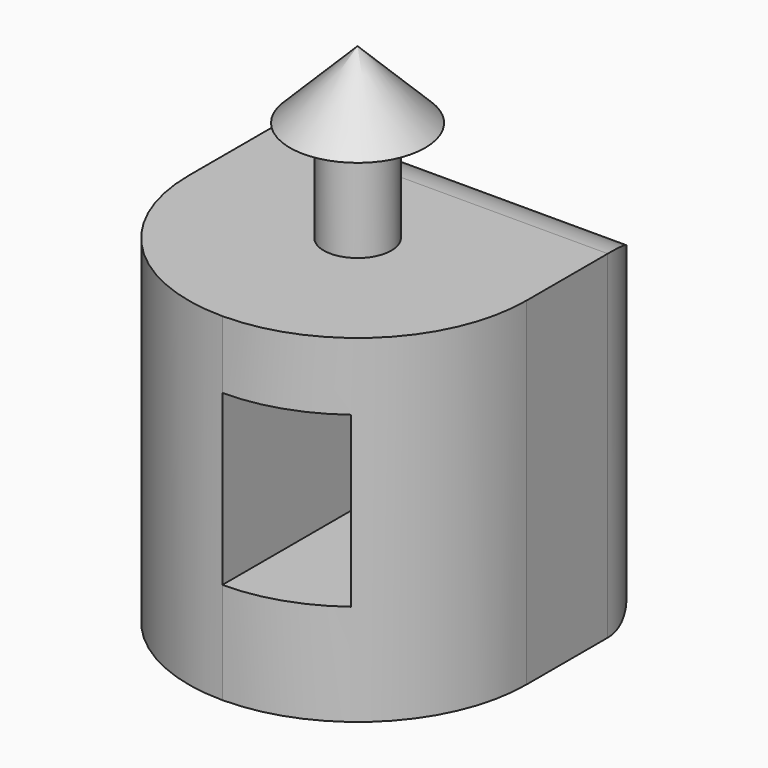
from build123d import *

# Parameters (mm, degrees)
F0_W          = 25.4
F0_H          = 25.4
F1_DEPTH      = 25.4
F2_T1_DEPTH   = 88.9
F3_R          = 2.54
F4_DEPTH      = 7.62
F5_R          = 5.08
F6_DEPTH      = 5.08
F7_SIZE       = 5.07999
F8_W          = 7.62
F8_H          = 12.7
F9_DEPTH      = 25.4
F10_T1_DEPTH  = 50.8
F10_T3_DEPTH  = 50.8
F10_T5_DEPTH  = 7.62
F10_T7_DEPTH  = 12.7
F10_T13_DEPTH = 20.32
F10_T18_DEPTH = 25.4
F10_T26_DEPTH = 20.32
F10_T30_DEPTH = 25.4
F10_T38_DEPTH = 25.4
F10_T43_DEPTH = 20.32
F10_T51_DEPTH = 20.32
F10_T55_DEPTH = 25.4


# Not quite as in the source:
# - a fillet or chamfer that OpenCascade refuses, or shapes differently, is made with other operations: its cross-section is extruded or revolved along the edge and cut away or added
# - a fillet or chamfer is up to 0.001 mm smaller than in the source, because OpenCascade refuses the exact size


with BuildPart() as f1:
    # F0 (on Top) → F1 (new body)
    with BuildSketch(Plane.XY):
        with Locations((12.7, 12.7)):
            Rectangle(F0_W, F0_H)
    extrude(amount=F1_DEPTH)

    # F2: fillet of radius 12.7 on 2 edges, made by hand

    # F2_s2 → F2_t1 (cut)
    with BuildSketch(Plane.XY.offset(-31.75)):
        with BuildLine():
            ThreePointArc((0, 12.7), (3.7197438789, 3.7197438789), (12.7, 0))
            Line((12.7, 0), (0, 0))
            Line((0, 0), (0, 12.7))
        make_face()
        with BuildLine():
            ThreePointArc((12.7, 0), (21.6802561211, 3.7197438789), (25.4, 12.7))
            Line((25.4, 12.7), (25.4, 0))
            Line((25.4, 0), (12.7, 0))
        make_face()
    extrude(amount=F2_T1_DEPTH, mode=Mode.SUBTRACT)

    # F3 (on face) → F4 (join)
    with BuildSketch(Plane.XY.offset(25.4)):
        with Locations((12.7, 12.7)):
            Circle(F3_R)
    extrude(amount=F4_DEPTH)

    # F5 (on face) → F6 (join)
    with BuildSketch(Plane.XY.offset(33.02)):
        with Locations((12.7, 12.7)):
            Circle(F5_R)
    extrude(amount=F6_DEPTH)

    # F7 (size 5.08 in the source; OpenCascade refuses exactly that, so slightly less here)
    f7_edges = [f1.edges().sort_by_distance(p)[0] for p in [
        (7.62, 12.7, 38.1),
    ]]
    chamfer(f7_edges, length=F7_SIZE)

    # F8 (on face) → F9 (cut)
    with BuildSketch(Plane(origin=(0, 25.4, 0), x_dir=(-1, 0, 0), z_dir=(0, 1, 0))):
        with Locations((-16.51, 13.97)):
            Rectangle(F8_W, F8_H)
    extrude(amount=-F9_DEPTH, mode=Mode.SUBTRACT)

    # F10: fillet of radius 5.08 on 8 edges, made by hand

    # F10_s2 → F10_t1 (cut)
    with BuildSketch(Plane.XY.offset(-12.7)):
        with BuildLine():
            ThreePointArc((20.32, 25.4), (23.9121024484, 23.9121024484), (25.4, 20.32))
            Line((25.4, 20.32), (25.4, 25.4))
            Line((25.4, 25.4), (20.32, 25.4))
        make_face()
        with BuildLine():
            ThreePointArc((5.08, 25.4), (1.4878975516, 23.9121024484), (0, 20.32))
            Line((0, 20.32), (0, 25.4))
            Line((0, 25.4), (5.08, 25.4))
        make_face()
    extrude(amount=F10_T1_DEPTH, mode=Mode.SUBTRACT)

    # F10_s4 → F10_t3 (cut)
    with BuildSketch(Plane.YZ.offset(-12.7)):
        with BuildLine():
            ThreePointArc((25.4, 5.08), (23.9121024484, 1.4878975516), (20.32, 0))
            Line((20.32, 0), (25.4, 0))
            Line((25.4, 0), (25.4, 5.08))
        make_face()
        with BuildLine():
            ThreePointArc((20.32, 25.4), (23.9121024484, 23.9121024484), (25.4, 20.32))
            Line((25.4, 20.32), (25.4, 25.4))
            Line((25.4, 25.4), (20.32, 25.4))
        make_face()
    extrude(amount=F10_T3_DEPTH, mode=Mode.SUBTRACT)

    # F10_s6 → F10_t5 (cut)
    with BuildSketch(Plane.YZ.offset(12.7)):
        with BuildLine():
            ThreePointArc((25.4, 2.54), (23.9121024484, 6.1321024484), (20.32, 7.62))
            Line((20.32, 7.62), (25.4, 7.62))
            Line((25.4, 7.62), (25.4, 2.54))
        make_face()
        with BuildLine():
            ThreePointArc((25.4, 25.4), (23.9121024484, 21.8078975516), (20.32, 20.32))
            Line((20.32, 20.32), (25.4, 20.32))
            Line((25.4, 20.32), (25.4, 25.4))
        make_face()
    extrude(amount=F10_T5_DEPTH, mode=Mode.SUBTRACT)

    # F10_s8 → F10_t7 (cut)
    with BuildSketch(Plane.XY.offset(7.62)):
        with BuildLine():
            ThreePointArc((25.4, 25.4), (21.8078975516, 23.9121024484), (20.32, 20.32))
            Line((20.32, 20.32), (20.32, 25.4))
            Line((20.32, 25.4), (25.4, 25.4))
        make_face()
        with BuildLine():
            ThreePointArc((7.62, 25.4), (11.2121024484, 23.9121024484), (12.7, 20.32))
            Line((12.7, 20.32), (12.7, 25.4))
            Line((12.7, 25.4), (7.62, 25.4))
        make_face()
    extrude(amount=F10_T7_DEPTH, mode=Mode.SUBTRACT)


with BuildPart() as f10_tool11:
    # F10_s12 → F10_t13 (new body)
    with BuildSketch(Plane.YZ.offset(33.02)):
        with BuildLine():
            ThreePointArc((25.4, 2.54), (23.9121024484, 6.1321024484), (20.32, 7.62))
            Line((20.32, 7.62), (25.4, 7.62))
            Line((25.4, 7.62), (25.4, 2.54))
        make_face()
    extrude(amount=-F10_T13_DEPTH)

    split(bisect_by=Plane.YZ.offset(25.4), keep=Keep.BOTTOM)

    split(bisect_by=Plane.YZ.offset(20.32), keep=Keep.TOP)


with BuildPart() as f10_tool16:
    # F10_s17 → F10_t18 (new body)
    with BuildSketch(Plane.XY.offset(20.32)):
        with BuildLine():
            ThreePointArc((25.4, 25.4), (21.8078975516, 23.9121024484), (20.32, 20.32))
            Line((20.32, 20.32), (20.32, 25.4))
            Line((20.32, 25.4), (25.4, 25.4))
        make_face()
    extrude(amount=-F10_T18_DEPTH)

    split(bisect_by=Plane.XY, keep=Keep.TOP)

    split(bisect_by=Plane.XY.offset(7.62), keep=Keep.BOTTOM)


with BuildPart() as f10_tool11_1:
    add(f10_tool11.part)

    # F10_t21: intersect F10_tool16
    add(f10_tool16.part, mode=Mode.INTERSECT)


with BuildPart() as f1_1:
    add(f1.part)

    # F10_t9: cut F10_tool11
    add(f10_tool11_1.part, mode=Mode.SUBTRACT)


with BuildPart() as f10_tool24:
    # F10_s25 → F10_t26 (new body)
    with BuildSketch(Plane.YZ.offset(20.32)):
        with BuildLine():
            ThreePointArc((25.4, 2.54), (23.9121024484, 6.1321024484), (20.32, 7.62))
            Line((20.32, 7.62), (25.4, 7.62))
            Line((25.4, 7.62), (25.4, 2.54))
        make_face()
    extrude(amount=-F10_T26_DEPTH)

    split(bisect_by=Plane.YZ.offset(12.7), keep=Keep.BOTTOM)


with BuildPart() as f10_tool28:
    # F10_s29 → F10_t30 (new body)
    with BuildSketch(Plane.XY.offset(-5.08)):
        with BuildLine():
            ThreePointArc((7.62, 25.4), (11.2121024484, 23.9121024484), (12.7, 20.32))
            Line((12.7, 20.32), (12.7, 25.4))
            Line((12.7, 25.4), (7.62, 25.4))
        make_face()
    extrude(amount=F10_T30_DEPTH)

    split(bisect_by=Plane.XY, keep=Keep.TOP)

    split(bisect_by=Plane.XY.offset(7.62), keep=Keep.BOTTOM)


with BuildPart() as f10_tool24_1:
    add(f10_tool24.part)

    # F10_t33: intersect F10_tool28
    add(f10_tool28.part, mode=Mode.INTERSECT)


with BuildPart() as f1_2:
    add(f1_1.part)

    # F10_t22: cut F10_tool24
    add(f10_tool24_1.part, mode=Mode.SUBTRACT)


with BuildPart() as f10_tool36:
    # F10_s37 → F10_t38 (new body)
    with BuildSketch(Plane.XY.offset(33.02)):
        with BuildLine():
            ThreePointArc((25.4, 25.4), (21.8078975516, 23.9121024484), (20.32, 20.32))
            Line((20.32, 20.32), (20.32, 25.4))
            Line((20.32, 25.4), (25.4, 25.4))
        make_face()
    extrude(amount=-F10_T38_DEPTH)

    split(bisect_by=Plane.XY.offset(25.4), keep=Keep.BOTTOM)

    split(bisect_by=Plane.XY.offset(20.32), keep=Keep.TOP)


with BuildPart() as f10_tool41:
    # F10_s42 → F10_t43 (new body)
    with BuildSketch(Plane.YZ.offset(12.7)):
        with BuildLine():
            ThreePointArc((25.4, 25.4), (23.9121024484, 21.8078975516), (20.32, 20.32))
            Line((20.32, 20.32), (25.4, 20.32))
            Line((25.4, 20.32), (25.4, 25.4))
        make_face()
    extrude(amount=F10_T43_DEPTH)

    split(bisect_by=Plane.YZ.offset(25.4), keep=Keep.BOTTOM)

    split(bisect_by=Plane.YZ.offset(20.32), keep=Keep.TOP)


with BuildPart() as f10_tool36_1:
    add(f10_tool36.part)

    # F10_t46: intersect F10_tool41
    add(f10_tool41.part, mode=Mode.INTERSECT)


with BuildPart() as f1_3:
    add(f1_2.part)

    # F10_t34: cut F10_tool36
    add(f10_tool36_1.part, mode=Mode.SUBTRACT)


with BuildPart() as f10_tool49:
    # F10_s50 → F10_t51 (new body)
    with BuildSketch(Plane.YZ):
        with BuildLine():
            ThreePointArc((25.4, 25.4), (23.9121024484, 21.8078975516), (20.32, 20.32))
            Line((20.32, 20.32), (25.4, 20.32))
            Line((25.4, 20.32), (25.4, 25.4))
        make_face()
    extrude(amount=F10_T51_DEPTH)

    split(bisect_by=Plane.YZ.offset(12.7), keep=Keep.BOTTOM)


with BuildPart() as f10_tool53:
    # F10_s54 → F10_t55 (new body)
    with BuildSketch(Plane.XY.offset(7.62)):
        with BuildLine():
            ThreePointArc((7.62, 25.4), (11.2121024484, 23.9121024484), (12.7, 20.32))
            Line((12.7, 20.32), (12.7, 25.4))
            Line((12.7, 25.4), (7.62, 25.4))
        make_face()
    extrude(amount=F10_T55_DEPTH)

    split(bisect_by=Plane.XY.offset(25.4), keep=Keep.BOTTOM)

    split(bisect_by=Plane.XY.offset(20.32), keep=Keep.TOP)


with BuildPart() as f10_tool49_1:
    add(f10_tool49.part)

    # F10_t58: intersect F10_tool53
    add(f10_tool53.part, mode=Mode.INTERSECT)


with BuildPart() as f1_4:
    add(f1_3.part)

    # F10_t47: cut F10_tool49
    add(f10_tool49_1.part, mode=Mode.SUBTRACT)


solid = f1_4.part
